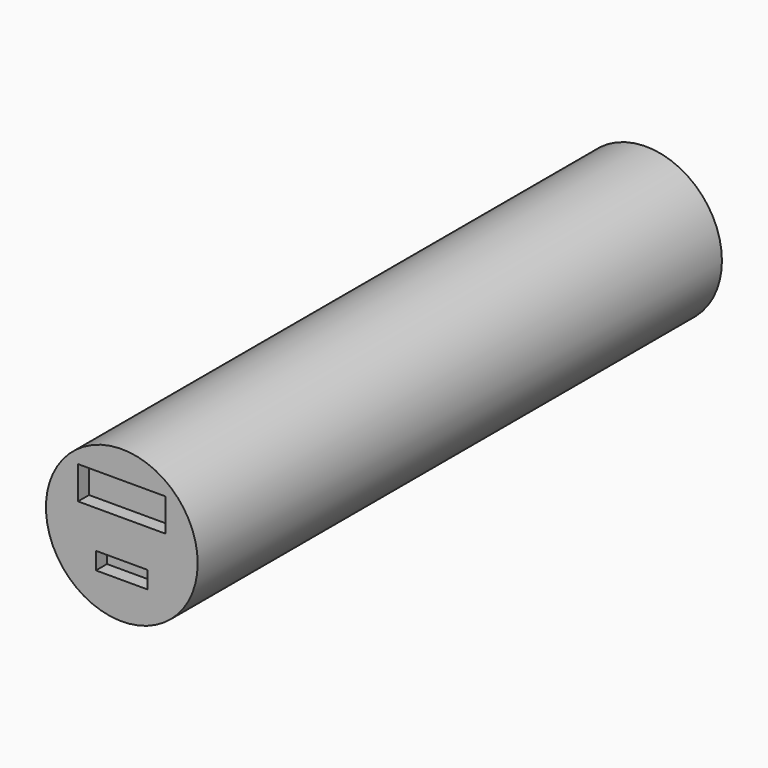
from build123d import *

# Parameters (mm, degrees)
F0_R     = 11
F1_DEPTH = 95
F2_W     = 12.7
F2_H     = 4.7625
F2_W_2   = 7.5
F2_H_2   = 2.5
F3_DEPTH = 2


# Not quite as in the source:
# - a feature names something its author has since deleted; it is built from what else it names


with BuildPart() as f1:
    # F0 (on Front) → F1 (new body)
    with BuildSketch(Plane.XZ):
        Circle(F0_R)
    extrude(amount=F1_DEPTH)

    # F2 (on face) → F3 (cut)
    with BuildSketch(Plane.XZ.offset(95)):
        with Locations((0, 4.6411268625)):
            Rectangle(F2_W, F2_H)
        with Locations((0, -4.4527297777)):
            Rectangle(F2_W_2, F2_H_2)
    extrude(amount=-F3_DEPTH, mode=Mode.SUBTRACT)


solid = f1.part
